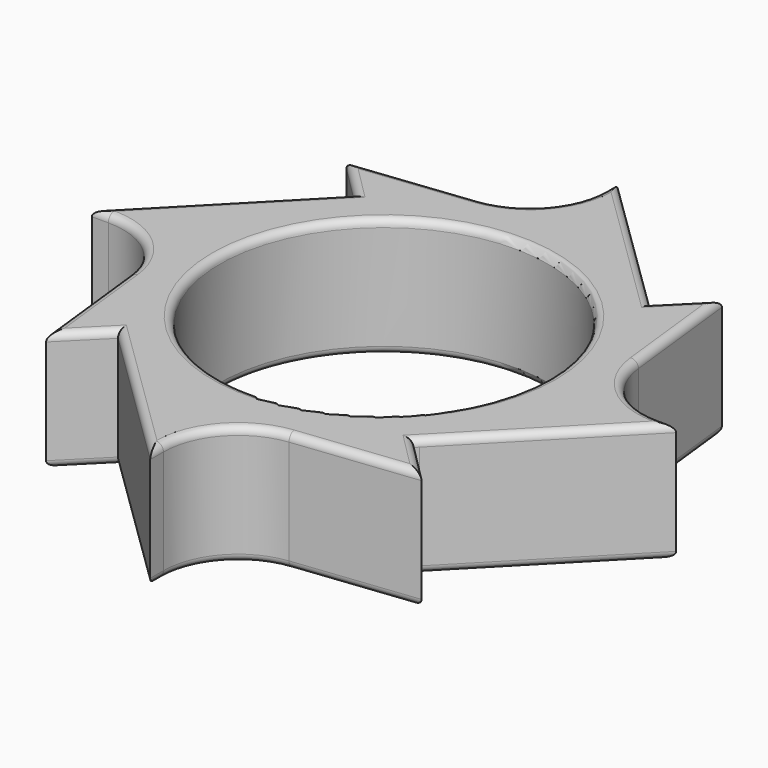
from build123d import *

# Parameters (mm, degrees)
F0_R          = 11
F1_DEPTH      = 8
F2_T1_DEPTH   = 2.3595992042
F2_T3_DEPTH   = 9.4400822056
F2_T5_DEPTH   = 2.3595992042
F2_T7_DEPTH   = 9.4400822056
F2_T9_DEPTH   = 2.3595992042
F2_T11_DEPTH  = 9.4400822056
F2_T13_DEPTH  = 2.3595992042
F2_T15_DEPTH  = 9.4400822056
F2_T18_ANGLE  = 83.5348176594
F2_T22_DEPTH  = 6.2837355468
F2_T27_DEPTH  = 16.3425213827
F2_T30_ANGLE  = 83.5348176594
F2_T34_DEPTH  = 6.2837355468
F2_T39_DEPTH  = 16.3425213827
F2_T42_ANGLE  = 83.5348176594
F2_T46_DEPTH  = 6.2837355468
F2_T51_DEPTH  = 16.3425213827
F2_T54_ANGLE  = 83.5348176594
F2_T58_DEPTH  = 6.2837355468
F2_T63_DEPTH  = 16.3425213827
F2_T68_ANGLE  = 83.5348176594
F2_T72_DEPTH  = 6.2837355468
F2_T77_DEPTH  = 16.3425213827
F2_T80_ANGLE  = 83.5348176594
F2_T84_DEPTH  = 6.2837355468
F2_T89_DEPTH  = 16.3425213827
F2_T92_ANGLE  = 83.5348176594
F2_T96_DEPTH  = 6.2837355468
F2_T101_DEPTH = 16.3425213827
F2_T104_ANGLE = 83.5348176594
F2_T108_DEPTH = 6.2837355468
F2_T113_DEPTH = 16.3425213827
F2_T121_DEPTH = 6.2837355468
F2_T125_DEPTH = 16.3425213827
F2_T132_DEPTH = 6.2837355468
F2_T136_DEPTH = 16.3425213827
F2_T143_DEPTH = 6.2837355468
F2_T147_DEPTH = 16.3425213827
F2_T154_DEPTH = 6.2837355468
F2_T158_DEPTH = 16.3425213827
F2_T165_DEPTH = 6.2837355468
F2_T169_DEPTH = 16.3425213827
F2_T176_DEPTH = 6.2837355468
F2_T180_DEPTH = 16.3425213827
F2_T187_DEPTH = 6.2837355468
F2_T191_DEPTH = 16.3425213827
F2_T198_DEPTH = 6.2837355468
F2_T202_DEPTH = 16.3425213827


# Not quite as in the source:
# - a fillet or chamfer that OpenCascade refuses, or shapes differently, is made with other operations: its cross-section is extruded or revolved along the edge and cut away or added


with BuildPart() as f1:
    # F0 (on Top) → F1 (new body)
    with BuildSketch(Plane.XY):
        with BuildLine():
            ThreePointArc((-85.174923351, 55.6713247205), (-75.4356150274, 59.7709133342), (-65.6050487553, 55.8952559455))
            Line((-65.6050487553, 55.8952559455), (-75.2754284143, 65.3468297839))
            Line((-75.2754284143, 65.3468297839), (-75.2754284143, 64.2372305797))
            ThreePointArc((-75.2754284143, 64.2372305797), (-76.5461533233, 60.9066889878), (-79.7124313324, 59.2690282604))
            Line((-79.7124313324, 59.2690282604), (-87.8504284143, 58.3468297839))
            Line((-87.8504284143, 58.3468297839), (-85.174923351, 55.6713247205))
        make_face()
        with BuildLine():
            ThreePointArc((-65.3759334777, 55.6713247205), (-62.3411149592, 51.129397837), (-61.2754284143, 45.7718297839))
            ThreePointArc((-61.2754284143, 45.7718297839), (-62.2806608854, 40.5626055741), (-65.1520022527, 36.1014501249))
            Line((-65.1520022527, 36.1014501249), (-55.7004284143, 45.7718297839))
            Line((-55.7004284143, 45.7718297839), (-56.8100276185, 45.7718297839))
            ThreePointArc((-56.8100276185, 45.7718297839), (-60.1405692104, 47.0425546929), (-61.7782299379, 50.208832702))
            Line((-61.7782299379, 50.208832702), (-62.7004284143, 58.3468297839))
            Line((-62.7004284143, 58.3468297839), (-65.3759334777, 55.6713247205))
        make_face()
        with BuildLine():
            Line((-62.7004284143, 33.1968297839), (-65.3759334777, 35.8723348473))
            ThreePointArc((-65.3759334777, 35.8723348473), (-75.1152418013, 31.7727462336), (-84.9458080734, 35.6484036223))
            Line((-84.9458080734, 35.6484036223), (-75.2754284143, 26.1968297839))
            Line((-75.2754284143, 26.1968297839), (-75.2754284143, 27.3064289881))
            ThreePointArc((-75.2754284143, 27.3064289881), (-74.0047035054, 30.63697058), (-70.8384254963, 32.2746313074))
            Line((-70.8384254963, 32.2746313074), (-62.7004284143, 33.1968297839))
        make_face()
        with BuildLine():
            ThreePointArc((-85.174923351, 35.8723348473), (-89.2745119647, 45.6116431709), (-85.398854576, 55.442209443))
            Line((-85.398854576, 55.442209443), (-94.8504284143, 45.7718297839))
            Line((-94.8504284143, 45.7718297839), (-93.7408292102, 45.7718297839))
            ThreePointArc((-93.7408292102, 45.7718297839), (-90.4102876183, 44.501104875), (-88.7726268908, 41.3348268658))
            Line((-88.7726268908, 41.3348268658), (-87.8504284143, 33.1968297839))
            Line((-87.8504284143, 33.1968297839), (-85.174923351, 35.8723348473))
        make_face()
        with BuildLine():
            ThreePointArc((-65.1520022527, 36.1014501249), (-62.2806608854, 40.5626055741), (-61.2754284143, 45.7718297839))
            ThreePointArc((-61.2754284143, 45.7718297839), (-62.3411149592, 51.129397837), (-65.3759334777, 55.6713247205))
            Line((-65.3759334777, 55.6713247205), (-65.6050487553, 55.8952559455))
            ThreePointArc((-65.6050487553, 55.8952559455), (-75.4356150274, 59.7709133342), (-85.174923351, 55.6713247205))
            Line((-85.174923351, 55.6713247205), (-85.398854576, 55.442209443))
            ThreePointArc((-85.398854576, 55.442209443), (-89.2745119647, 45.6116431709), (-85.174923351, 35.8723348473))
            Line((-85.174923351, 35.8723348473), (-84.9458080734, 35.6484036223))
            ThreePointArc((-84.9458080734, 35.6484036223), (-75.1152418013, 31.7727462336), (-65.3759334777, 35.8723348473))
            Line((-65.3759334777, 35.8723348473), (-65.1520022527, 36.1014501249))
        make_face()
        with Locations((-75.2754284143, 45.7718297839)):
            Circle(F0_R, mode=Mode.SUBTRACT)
    extrude(amount=F1_DEPTH)

    # F2: fillet of radius 0.5 on 42 edges, made by hand

    # F2_s2 → F2_t1 (cut)
    with BuildSketch(Plane.XZ.offset(-66.5968297839)):
        with BuildLine():
            ThreePointArc((-75.2754284143, 7.5), (-75.1289818049, 7.8535533906), (-74.7754284143, 8))
            Line((-74.7754284143, 8), (-75.2754284143, 8))
            Line((-75.2754284143, 8), (-75.2754284143, 7.5))
        make_face()
        with BuildLine():
            ThreePointArc((-75.2754284143, 0.5), (-75.1289818049, 0.1464466094), (-74.7754284143, 0))
            Line((-74.7754284143, 0), (-75.2754284143, 0))
            Line((-75.2754284143, 0), (-75.2754284143, 0.5))
        make_face()
    extrude(amount=F2_T1_DEPTH, mode=Mode.SUBTRACT)

    # F2_s4 → F2_t3 (cut)
    with BuildSketch(Plane(origin=(-72.0705704007, -8.1670427691, 0), x_dir=(0, 0, 1), z_dir=(-0.9936404639, -0.1125994164, 0))):
        with BuildLine():
            ThreePointArc((7.5, 67.86767798), (7.8535533906, 67.7212313705), (8, 67.36767798))
            Line((8, 67.36767798), (8, 67.86767798))
            Line((8, 67.86767798), (7.5, 67.86767798))
        make_face()
        with BuildLine():
            ThreePointArc((0.5, 67.86767798), (0.1464466094, 67.7212313705), (0, 67.36767798))
            Line((0, 67.36767798), (0, 67.86767798))
            Line((0, 67.86767798), (0.5, 67.86767798))
        make_face()
    extrude(amount=F2_T3_DEPTH, mode=Mode.SUBTRACT)

    # F2_s6 → F2_t5 (cut)
    with BuildSketch(Plane.YZ.offset(-96.1004284143)):
        with BuildLine():
            ThreePointArc((45.7718297839, 7.5), (45.9182763933, 7.8535533906), (46.2718297839, 8))
            Line((46.2718297839, 8), (45.7718297839, 8))
            Line((45.7718297839, 8), (45.7718297839, 7.5))
        make_face()
        with BuildLine():
            ThreePointArc((45.7718297839, 0.5), (45.9182763933, 0.1464466094), (46.2718297839, 0))
            Line((46.2718297839, 0), (45.7718297839, 0))
            Line((45.7718297839, 0), (45.7718297839, 0.5))
        make_face()
    extrude(amount=F2_T5_DEPTH, mode=Mode.SUBTRACT)

    # F2_s8 → F2_t7 (cut)
    with BuildSketch(Plane(origin=(-5.7501934997, 50.7429356199, 0), x_dir=(0, 0, 1), z_dir=(0.1125994164, -0.9936404639, 0))):
        with BuildLine():
            ThreePointArc((7.5, 83.553796781), (7.8535533906, 83.4073501716), (8, 83.053796781))
            Line((8, 83.053796781), (8, 83.553796781))
            Line((8, 83.553796781), (7.5, 83.553796781))
        make_face()
        with BuildLine():
            ThreePointArc((0.5, 83.553796781), (0.1464466094, 83.4073501716), (0, 83.053796781))
            Line((0, 83.053796781), (0, 83.553796781))
            Line((0, 83.553796781), (0.5, 83.553796781))
        make_face()
    extrude(amount=F2_T7_DEPTH, mode=Mode.SUBTRACT)

    # F2_s10 → F2_t9 (cut)
    with BuildSketch(Plane.XZ.offset(-27.3064289881)):
        with BuildLine():
            ThreePointArc((-75.2754284143, 7.5), (-75.4218750238, 7.8535533906), (-75.7754284143, 8))
            Line((-75.7754284143, 8), (-75.2754284143, 8))
            Line((-75.2754284143, 8), (-75.2754284143, 7.5))
        make_face()
        with BuildLine():
            ThreePointArc((-75.2754284143, 0.5), (-75.4218750238, 0.1464466094), (-75.7754284143, 0))
            Line((-75.7754284143, 0), (-75.2754284143, 0))
            Line((-75.2754284143, 0), (-75.2754284143, 0.5))
        make_face()
    extrude(amount=F2_T9_DEPTH, mode=Mode.SUBTRACT)

    # F2_s12 → F2_t11 (cut)
    with BuildSketch(Plane(origin=(-66.3292979816, -7.516441322, 0), x_dir=(0, 0, 1), z_dir=(0.9936404639, 0.1125994164, 0))):
        with BuildLine():
            ThreePointArc((7.5, -40.0457449917), (7.8535533906, -40.1921916011), (8, -40.5457449917))
            Line((8, -40.5457449917), (8, -40.0457449917))
            Line((8, -40.0457449917), (7.5, -40.0457449917))
        make_face()
        with BuildLine():
            ThreePointArc((0.5, -40.0457449917), (0.1464466094, -40.1921916011), (0, -40.5457449917))
            Line((0, -40.5457449917), (0, -40.0457449917))
            Line((0, -40.0457449917), (0.5, -40.0457449917))
        make_face()
    extrude(amount=F2_T11_DEPTH, mode=Mode.SUBTRACT)

    # F2_s14 → F2_t13 (cut)
    with BuildSketch(Plane.YZ.offset(-56.8100276185)):
        with BuildLine():
            ThreePointArc((45.7718297839, 7.5), (45.6253831745, 7.8535533906), (45.2718297839, 8))
            Line((45.2718297839, 8), (45.7718297839, 8))
            Line((45.7718297839, 8), (45.7718297839, 7.5))
        make_face()
        with BuildLine():
            ThreePointArc((45.7718297839, 0.5), (45.6253831745, 0.1464466094), (45.2718297839, 0))
            Line((45.2718297839, 0), (45.7718297839, 0))
            Line((45.7718297839, 0), (45.7718297839, 0.5))
        make_face()
    extrude(amount=F2_T13_DEPTH, mode=Mode.SUBTRACT)

    # F2_s16 → F2_t15 (cut)
    with BuildSketch(Plane(origin=(-6.4007949468, 56.484208039, 0), x_dir=(0, 0, 1), z_dir=(-0.1125994164, 0.9936404639, 0))):
        with BuildLine():
            ThreePointArc((7.5, -55.7318637928), (7.8535533906, -55.8783104022), (8, -56.2318637928))
            Line((8, -56.2318637928), (8, -55.7318637928))
            Line((8, -55.7318637928), (7.5, -55.7318637928))
        make_face()
        with BuildLine():
            ThreePointArc((0.5, -55.7318637928), (0.1464466094, -55.8783104022), (0, -56.2318637928))
            Line((0, -56.2318637928), (0, -55.7318637928))
            Line((0, -55.7318637928), (0.5, -55.7318637928))
        make_face()
    extrude(amount=F2_T15_DEPTH, mode=Mode.SUBTRACT)

    # F2_s17 → F2_t18 (revolve, cut)
    with BuildSketch(Plane.XZ.offset(-64.2372305797)):
        with BuildLine():
            ThreePointArc((-75.2754284143, 7.5), (-75.1289818049, 7.8535533906), (-74.7754284143, 8))
            Line((-74.7754284143, 8), (-75.2754284143, 8))
            Line((-75.2754284143, 8), (-75.2754284143, 7.5))
        make_face()
    revolve(axis=Axis((-80.2754284143, 64.2372305797, 8), (0, 0, -1)), revolution_arc=F2_T18_ANGLE, mode=Mode.SUBTRACT)


with BuildPart() as f2_tool20:
    # F2_s21 → F2_t22 (new body)
    with BuildSketch(Plane(origin=(-73.9825125756, 73.9825125756, 0), x_dir=(0, 0, 1), z_dir=(0.7071067812, -0.7071067812, 0))):
        with BuildLine():
            ThreePointArc((7.5, 20.862194661), (7.8535533906, 20.7157480516), (8, 20.362194661))
            Line((8, 20.362194661), (8, 20.862194661))
            Line((8, 20.862194661), (7.5, 20.862194661))
        make_face()
    extrude(amount=F2_T22_DEPTH)

    split(bisect_by=Plane(origin=(-71.3903349466, 69.7750290975, 0), x_dir=(0, 0, 1), z_dir=(-0.7151511392, 0.6989698478, 0)), keep=Keep.TOP)


with BuildPart() as f1_1:
    add(f1.part)

    # F2_t19: cut F2_tool20
    add(f2_tool20.part, mode=Mode.SUBTRACT)


with BuildPart() as f2_tool25:
    # F2_s26 → F2_t27 (new body)
    with BuildSketch(Plane(origin=(-12.9108760947, -13.209765453, 0), x_dir=(0, 0, 1), z_dir=(-0.6989698478, -0.7151511392, 0))):
        with BuildLine():
            ThreePointArc((7.5, 99.8255208318), (7.8535533906, 99.6790742224), (8, 99.3255208318))
            Line((8, 99.3255208318), (8, 99.8255208318))
            Line((8, 99.8255208318), (7.5, 99.8255208318))
        make_face()
    extrude(amount=F2_T27_DEPTH)

    split(bisect_by=Plane(origin=(-14.7517993152, -14.7517993152, 0), x_dir=(0, 0, 1), z_dir=(-0.7071067812, -0.7071067812, 0)), keep=Keep.TOP)


with BuildPart() as f1_2:
    add(f1_1.part)

    # F2_t24: cut F2_tool25
    add(f2_tool25.part, mode=Mode.SUBTRACT)

    # F2_s29 → F2_t30 (revolve, cut)
    with BuildSketch(Plane.YZ.offset(-93.7408292102)):
        with BuildLine():
            ThreePointArc((45.7718297839, 7.5), (45.9182763933, 7.8535533906), (46.2718297839, 8))
            Line((46.2718297839, 8), (45.7718297839, 8))
            Line((45.7718297839, 8), (45.7718297839, 7.5))
        make_face()
    revolve(axis=Axis((-93.7408292102, 40.7718297839, 8), (0, 0, -1)), revolution_arc=F2_T30_ANGLE, mode=Mode.SUBTRACT)


with BuildPart() as f2_tool32:
    # F2_s33 → F2_t34 (new body)
    with BuildSketch(Plane(origin=(-28.2106827917, -28.2106827917, 0), x_dir=(0, 0, 1), z_dir=(0.7071067812, 0.7071067812, 0))):
        with BuildLine():
            ThreePointArc((7.5, -85.593337116), (7.8535533906, -85.7397837254), (8, -86.093337116))
            Line((8, -86.093337116), (8, -85.593337116))
            Line((8, -85.593337116), (7.5, -85.593337116))
        make_face()
    extrude(amount=F2_T34_DEPTH)

    split(bisect_by=Plane(origin=(-23.6814913147, -24.2297225649, 0), x_dir=(0, 0, 1), z_dir=(-0.6989698478, -0.7151511392, 0)), keep=Keep.TOP)


with BuildPart() as f1_3:
    add(f1_2.part)

    # F2_t31: cut F2_tool32
    add(f2_tool32.part, mode=Mode.SUBTRACT)


with BuildPart() as f2_tool37:
    # F2_s38 → F2_t39 (new body)
    with BuildSketch(Plane(origin=(-62.3873709603, 60.9757697219, 0), x_dir=(0, 0, 1), z_dir=(0.7151511392, -0.6989698478, 0))):
        with BuildLine():
            ThreePointArc((7.5, 33.8805620741), (7.8535533906, 33.7341154647), (8, 33.3805620741))
            Line((8, 33.3805620741), (8, 33.8805620741))
            Line((8, 33.8805620741), (7.5, 33.8805620741))
        make_face()
    extrude(amount=F2_T39_DEPTH)

    split(bisect_by=Plane(origin=(-60.5236290991, 60.5236290991, 0), x_dir=(0, 0, 1), z_dir=(0.7071067812, -0.7071067812, 0)), keep=Keep.TOP)


with BuildPart() as f1_4:
    add(f1_3.part)

    # F2_t36: cut F2_tool37
    add(f2_tool37.part, mode=Mode.SUBTRACT)

    # F2_s41 → F2_t42 (revolve, cut)
    with BuildSketch(Plane.XZ.offset(-27.3064289881)):
        with BuildLine():
            ThreePointArc((-75.2754284143, 7.5), (-75.4218750238, 7.8535533906), (-75.7754284143, 8))
            Line((-75.7754284143, 8), (-75.2754284143, 8))
            Line((-75.2754284143, 8), (-75.2754284143, 7.5))
        make_face()
    revolve(axis=Axis((-70.2754284143, 27.3064289881, 8), (0, 0, -1)), revolution_arc=F2_T42_ANGLE, mode=Mode.SUBTRACT)


with BuildPart() as f2_tool44:
    # F2_s45 → F2_t46 (new body)
    with BuildSketch(Plane(origin=(-47.0647456226, 47.0647456226, 0), x_dir=(0, 0, 1), z_dir=(-0.7071067812, 0.7071067812, 0))):
        with BuildLine():
            ThreePointArc((7.5, -20.862194661), (7.8535533906, -21.0086412704), (8, -21.362194661))
            Line((8, -21.362194661), (8, -20.862194661))
            Line((8, -20.862194661), (7.5, -20.862194661))
        make_face()
    extrude(amount=F2_T46_DEPTH)

    split(bisect_by=Plane(origin=(-51.3674138484, 50.2051545019, 0), x_dir=(0, 0, 1), z_dir=(0.7151511392, -0.6989698478, 0)), keep=Keep.TOP)


with BuildPart() as f1_5:
    add(f1_4.part)

    # F2_t43: cut F2_tool44
    add(f2_tool44.part, mode=Mode.SUBTRACT)


with BuildPart() as f2_tool49:
    # F2_s50 → F2_t51 (new body)
    with BuildSketch(Plane(origin=(-14.8822319391, -15.2267585786, 0), x_dir=(0, 0, 1), z_dir=(0.6989698478, 0.7151511392, 0))):
        with BuildLine():
            ThreePointArc((7.5, -71.8273537312), (7.8535533906, -71.9738003406), (8, -72.3273537312))
            Line((8, -72.3273537312), (8, -71.8273537312))
            Line((8, -71.8273537312), (7.5, -71.8273537312))
        make_face()
    extrude(amount=F2_T51_DEPTH)

    split(bisect_by=Plane(origin=(-14.7517993152, -14.7517993152, 0), x_dir=(0, 0, 1), z_dir=(0.7071067812, 0.7071067812, 0)), keep=Keep.TOP)


with BuildPart() as f1_6:
    add(f1_5.part)

    # F2_t48: cut F2_tool49
    add(f2_tool49.part, mode=Mode.SUBTRACT)

    # F2_s53 → F2_t54 (revolve, cut)
    with BuildSketch(Plane.YZ.offset(-56.8100276185)):
        with BuildLine():
            ThreePointArc((45.7718297839, 7.5), (45.6253831745, 7.8535533906), (45.2718297839, 8))
            Line((45.2718297839, 8), (45.7718297839, 8))
            Line((45.7718297839, 8), (45.7718297839, 7.5))
        make_face()
    revolve(axis=Axis((-56.8100276185, 50.7718297839, 8), (0, 0, -1)), revolution_arc=F2_T54_ANGLE, mode=Mode.SUBTRACT)


with BuildPart() as f2_tool56:
    # F2_s57 → F2_t58 (new body)
    with BuildSketch(Plane(origin=(-1.2929158387, -1.2929158387, 0), x_dir=(0, 0, 1), z_dir=(-0.7071067812, -0.7071067812, 0))):
        with BuildLine():
            ThreePointArc((7.5, 85.593337116), (7.8535533906, 85.4468905066), (8, 85.093337116))
            Line((8, 85.093337116), (8, 85.593337116))
            Line((8, 85.593337116), (7.5, 85.593337116))
        make_face()
    extrude(amount=F2_T58_DEPTH)

    split(bisect_by=Plane(origin=(-4.111616719, -4.2068014667, 0), x_dir=(0, 0, 1), z_dir=(0.6989698478, 0.7151511392, 0)), keep=Keep.TOP)


with BuildPart() as f1_7:
    add(f1_6.part)

    # F2_t55: cut F2_tool56
    add(f2_tool56.part, mode=Mode.SUBTRACT)


with BuildPart() as f2_tool61:
    # F2_s62 → F2_t63 (new body)
    with BuildSketch(Plane(origin=(-60.3703778347, 59.0044138775, 0), x_dir=(0, 0, 1), z_dir=(-0.7151511392, 0.6989698478, 0))):
        with BuildLine():
            ThreePointArc((7.5, -5.8823949735), (7.8535533906, -6.0288415829), (8, -6.3823949735))
            Line((8, -6.3823949735), (8, -5.8823949735))
            Line((8, -5.8823949735), (7.5, -5.8823949735))
        make_face()
    extrude(amount=F2_T63_DEPTH)

    split(bisect_by=Plane(origin=(-60.5236290991, 60.5236290991, 0), x_dir=(0, 0, 1), z_dir=(-0.7071067812, 0.7071067812, 0)), keep=Keep.TOP)


with BuildPart() as f1_8:
    add(f1_7.part)

    # F2_t60: cut F2_tool61
    add(f2_tool61.part, mode=Mode.SUBTRACT)

    # F2_s65 → F2_t66 (revolve, cut)
    with BuildSketch(Plane.XZ.offset(-45.7718297839)):
        with BuildLine():
            ThreePointArc((-64.2754284143, 7.5), (-64.1289818049, 7.8535533906), (-63.7754284143, 8))
            Line((-63.7754284143, 8), (-64.2754284143, 8))
            Line((-64.2754284143, 8), (-64.2754284143, 7.5))
        make_face()
    revolve(axis=Axis((-75.2754284143, 45.7718297839, 8), (0, 0, 1)), mode=Mode.SUBTRACT)

    # F2_s67 → F2_t68 (revolve, cut)
    with BuildSketch(Plane.XZ.offset(-64.2372305797)):
        with BuildLine():
            ThreePointArc((-75.2754284143, 0.5), (-75.1289818049, 0.1464466094), (-74.7754284143, 0))
            Line((-74.7754284143, 0), (-75.2754284143, 0))
            Line((-75.2754284143, 0), (-75.2754284143, 0.5))
        make_face()
    revolve(axis=Axis((-80.2754284143, 64.2372305797, 0), (0, 0, -1)), revolution_arc=F2_T68_ANGLE, mode=Mode.SUBTRACT)


with BuildPart() as f2_tool70:
    # F2_s71 → F2_t72 (new body)
    with BuildSketch(Plane(origin=(-73.9825125756, 73.9825125756, 0), x_dir=(0, 0, 1), z_dir=(0.7071067812, -0.7071067812, 0))):
        with BuildLine():
            ThreePointArc((0.5, 20.862194661), (0.1464466094, 20.7157480516), (0, 20.362194661))
            Line((0, 20.362194661), (0, 20.862194661))
            Line((0, 20.862194661), (0.5, 20.862194661))
        make_face()
    extrude(amount=F2_T72_DEPTH)

    split(bisect_by=Plane(origin=(-71.3903349466, 69.7750290975, 0), x_dir=(0, 0, 1), z_dir=(-0.7151511392, 0.6989698478, 0)), keep=Keep.TOP)


with BuildPart() as f1_9:
    add(f1_8.part)

    # F2_t69: cut F2_tool70
    add(f2_tool70.part, mode=Mode.SUBTRACT)


with BuildPart() as f2_tool75:
    # F2_s76 → F2_t77 (new body)
    with BuildSketch(Plane(origin=(-12.9108760947, -13.209765453, 0), x_dir=(0, 0, 1), z_dir=(-0.6989698478, -0.7151511392, 0))):
        with BuildLine():
            ThreePointArc((0.5, 99.8255208318), (0.1464466094, 99.6790742224), (0, 99.3255208318))
            Line((0, 99.3255208318), (0, 99.8255208318))
            Line((0, 99.8255208318), (0.5, 99.8255208318))
        make_face()
    extrude(amount=F2_T77_DEPTH)

    split(bisect_by=Plane(origin=(-14.7517993152, -14.7517993152, 0), x_dir=(0, 0, 1), z_dir=(-0.7071067812, -0.7071067812, 0)), keep=Keep.TOP)


with BuildPart() as f1_10:
    add(f1_9.part)

    # F2_t74: cut F2_tool75
    add(f2_tool75.part, mode=Mode.SUBTRACT)

    # F2_s79 → F2_t80 (revolve, cut)
    with BuildSketch(Plane.YZ.offset(-93.7408292102)):
        with BuildLine():
            ThreePointArc((45.7718297839, 0.5), (45.9182763933, 0.1464466094), (46.2718297839, 0))
            Line((46.2718297839, 0), (45.7718297839, 0))
            Line((45.7718297839, 0), (45.7718297839, 0.5))
        make_face()
    revolve(axis=Axis((-93.7408292102, 40.7718297839, 0), (0, 0, -1)), revolution_arc=F2_T80_ANGLE, mode=Mode.SUBTRACT)


with BuildPart() as f2_tool82:
    # F2_s83 → F2_t84 (new body)
    with BuildSketch(Plane(origin=(-28.2106827917, -28.2106827917, 0), x_dir=(0, 0, 1), z_dir=(0.7071067812, 0.7071067812, 0))):
        with BuildLine():
            ThreePointArc((0.5, -85.593337116), (0.1464466094, -85.7397837254), (0, -86.093337116))
            Line((0, -86.093337116), (0, -85.593337116))
            Line((0, -85.593337116), (0.5, -85.593337116))
        make_face()
    extrude(amount=F2_T84_DEPTH)

    split(bisect_by=Plane(origin=(-23.6814913147, -24.2297225649, 0), x_dir=(0, 0, 1), z_dir=(-0.6989698478, -0.7151511392, 0)), keep=Keep.TOP)


with BuildPart() as f1_11:
    add(f1_10.part)

    # F2_t81: cut F2_tool82
    add(f2_tool82.part, mode=Mode.SUBTRACT)


with BuildPart() as f2_tool87:
    # F2_s88 → F2_t89 (new body)
    with BuildSketch(Plane(origin=(-62.3873709603, 60.9757697219, 0), x_dir=(0, 0, 1), z_dir=(0.7151511392, -0.6989698478, 0))):
        with BuildLine():
            ThreePointArc((0.5, 33.8805620741), (0.1464466094, 33.7341154647), (0, 33.3805620741))
            Line((0, 33.3805620741), (0, 33.8805620741))
            Line((0, 33.8805620741), (0.5, 33.8805620741))
        make_face()
    extrude(amount=F2_T89_DEPTH)

    split(bisect_by=Plane(origin=(-60.5236290991, 60.5236290991, 0), x_dir=(0, 0, 1), z_dir=(0.7071067812, -0.7071067812, 0)), keep=Keep.TOP)


with BuildPart() as f1_12:
    add(f1_11.part)

    # F2_t86: cut F2_tool87
    add(f2_tool87.part, mode=Mode.SUBTRACT)

    # F2_s91 → F2_t92 (revolve, cut)
    with BuildSketch(Plane.XZ.offset(-27.3064289881)):
        with BuildLine():
            ThreePointArc((-75.2754284143, 0.5), (-75.4218750238, 0.1464466094), (-75.7754284143, 0))
            Line((-75.7754284143, 0), (-75.2754284143, 0))
            Line((-75.2754284143, 0), (-75.2754284143, 0.5))
        make_face()
    revolve(axis=Axis((-70.2754284143, 27.3064289881, 0), (0, 0, -1)), revolution_arc=F2_T92_ANGLE, mode=Mode.SUBTRACT)


with BuildPart() as f2_tool94:
    # F2_s95 → F2_t96 (new body)
    with BuildSketch(Plane(origin=(-47.0647456226, 47.0647456226, 0), x_dir=(0, 0, 1), z_dir=(-0.7071067812, 0.7071067812, 0))):
        with BuildLine():
            ThreePointArc((0.5, -20.862194661), (0.1464466094, -21.0086412704), (0, -21.362194661))
            Line((0, -21.362194661), (0, -20.862194661))
            Line((0, -20.862194661), (0.5, -20.862194661))
        make_face()
    extrude(amount=F2_T96_DEPTH)

    split(bisect_by=Plane(origin=(-51.3674138484, 50.2051545019, 0), x_dir=(0, 0, 1), z_dir=(0.7151511392, -0.6989698478, 0)), keep=Keep.TOP)


with BuildPart() as f1_13:
    add(f1_12.part)

    # F2_t93: cut F2_tool94
    add(f2_tool94.part, mode=Mode.SUBTRACT)


with BuildPart() as f2_tool99:
    # F2_s100 → F2_t101 (new body)
    with BuildSketch(Plane(origin=(-14.8822319391, -15.2267585786, 0), x_dir=(0, 0, 1), z_dir=(0.6989698478, 0.7151511392, 0))):
        with BuildLine():
            ThreePointArc((0.5, -71.8273537312), (0.1464466094, -71.9738003406), (0, -72.3273537312))
            Line((0, -72.3273537312), (0, -71.8273537312))
            Line((0, -71.8273537312), (0.5, -71.8273537312))
        make_face()
    extrude(amount=F2_T101_DEPTH)

    split(bisect_by=Plane(origin=(-14.7517993152, -14.7517993152, 0), x_dir=(0, 0, 1), z_dir=(0.7071067812, 0.7071067812, 0)), keep=Keep.TOP)


with BuildPart() as f1_14:
    add(f1_13.part)

    # F2_t98: cut F2_tool99
    add(f2_tool99.part, mode=Mode.SUBTRACT)

    # F2_s103 → F2_t104 (revolve, cut)
    with BuildSketch(Plane.YZ.offset(-56.8100276185)):
        with BuildLine():
            ThreePointArc((45.7718297839, 0.5), (45.6253831745, 0.1464466094), (45.2718297839, 0))
            Line((45.2718297839, 0), (45.7718297839, 0))
            Line((45.7718297839, 0), (45.7718297839, 0.5))
        make_face()
    revolve(axis=Axis((-56.8100276185, 50.7718297839, 0), (0, 0, -1)), revolution_arc=F2_T104_ANGLE, mode=Mode.SUBTRACT)


with BuildPart() as f2_tool106:
    # F2_s107 → F2_t108 (new body)
    with BuildSketch(Plane(origin=(-1.2929158387, -1.2929158387, 0), x_dir=(0, 0, 1), z_dir=(-0.7071067812, -0.7071067812, 0))):
        with BuildLine():
            ThreePointArc((0.5, 85.593337116), (0.1464466094, 85.4468905066), (0, 85.093337116))
            Line((0, 85.093337116), (0, 85.593337116))
            Line((0, 85.593337116), (0.5, 85.593337116))
        make_face()
    extrude(amount=F2_T108_DEPTH)

    split(bisect_by=Plane(origin=(-4.111616719, -4.2068014667, 0), x_dir=(0, 0, 1), z_dir=(0.6989698478, 0.7151511392, 0)), keep=Keep.TOP)


with BuildPart() as f1_15:
    add(f1_14.part)

    # F2_t105: cut F2_tool106
    add(f2_tool106.part, mode=Mode.SUBTRACT)


with BuildPart() as f2_tool111:
    # F2_s112 → F2_t113 (new body)
    with BuildSketch(Plane(origin=(-60.3703778347, 59.0044138775, 0), x_dir=(0, 0, 1), z_dir=(-0.7151511392, 0.6989698478, 0))):
        with BuildLine():
            ThreePointArc((0.5, -5.8823949735), (0.1464466094, -6.0288415829), (0, -6.3823949735))
            Line((0, -6.3823949735), (0, -5.8823949735))
            Line((0, -5.8823949735), (0.5, -5.8823949735))
        make_face()
    extrude(amount=F2_T113_DEPTH)

    split(bisect_by=Plane(origin=(-60.5236290991, 60.5236290991, 0), x_dir=(0, 0, 1), z_dir=(-0.7071067812, 0.7071067812, 0)), keep=Keep.TOP)


with BuildPart() as f1_16:
    add(f1_15.part)

    # F2_t110: cut F2_tool111
    add(f2_tool111.part, mode=Mode.SUBTRACT)

    # F2_s115 → F2_t116 (revolve, cut)
    with BuildSketch(Plane.XZ.offset(-45.7718297839)):
        with BuildLine():
            ThreePointArc((-64.2754284143, 0.5), (-64.1289818049, 0.1464466094), (-63.7754284143, 0))
            Line((-63.7754284143, 0), (-64.2754284143, 0))
            Line((-64.2754284143, 0), (-64.2754284143, 0.5))
        make_face()
    revolve(axis=Axis((-75.2754284143, 45.7718297839, 0), (0, 0, 1)), mode=Mode.SUBTRACT)


with BuildPart() as f2_tool119:
    # F2_s120 → F2_t121 (new body)
    with BuildSketch(Plane(origin=(-73.9825125756, 73.9825125756, 0), x_dir=(0, 0, 1), z_dir=(0.7071067812, -0.7071067812, 0))):
        with BuildLine():
            ThreePointArc((7.5, 20.862194661), (7.8535533906, 20.7157480516), (8, 20.362194661))
            Line((8, 20.362194661), (8, 20.862194661))
            Line((8, 20.862194661), (7.5, 20.862194661))
        make_face()
    extrude(amount=F2_T121_DEPTH)

    split(bisect_by=Plane(origin=(-71.3903349466, 69.7750290975, 0), x_dir=(0, 0, 1), z_dir=(0.7151511392, -0.6989698478, 0)), keep=Keep.TOP)


with BuildPart() as f2_tool123:
    # F2_s124 → F2_t125 (new body)
    with BuildSketch(Plane(origin=(-12.9108760947, -13.209765453, 0), x_dir=(0, 0, 1), z_dir=(-0.6989698478, -0.7151511392, 0))):
        with BuildLine():
            ThreePointArc((7.5, 99.8255208318), (7.8535533906, 99.6790742224), (8, 99.3255208318))
            Line((8, 99.3255208318), (8, 99.8255208318))
            Line((8, 99.8255208318), (7.5, 99.8255208318))
        make_face()
    extrude(amount=F2_T125_DEPTH)

    split(bisect_by=Plane(origin=(-14.7517993152, -14.7517993152, 0), x_dir=(0, 0, 1), z_dir=(0.7071067812, 0.7071067812, 0)), keep=Keep.TOP)


with BuildPart() as f2_tool119_1:
    add(f2_tool119.part)

    # F2_t127: intersect F2_tool123
    add(f2_tool123.part, mode=Mode.INTERSECT)


with BuildPart() as f1_17:
    add(f1_16.part)

    # F2_t117: cut F2_tool119
    add(f2_tool119_1.part, mode=Mode.SUBTRACT)


with BuildPart() as f2_tool130:
    # F2_s131 → F2_t132 (new body)
    with BuildSketch(Plane(origin=(-28.2106827917, -28.2106827917, 0), x_dir=(0, 0, 1), z_dir=(0.7071067812, 0.7071067812, 0))):
        with BuildLine():
            ThreePointArc((7.5, -85.593337116), (7.8535533906, -85.7397837254), (8, -86.093337116))
            Line((8, -86.093337116), (8, -85.593337116))
            Line((8, -85.593337116), (7.5, -85.593337116))
        make_face()
    extrude(amount=F2_T132_DEPTH)

    split(bisect_by=Plane(origin=(-23.6814913147, -24.2297225649, 0), x_dir=(0, 0, 1), z_dir=(0.6989698478, 0.7151511392, 0)), keep=Keep.TOP)


with BuildPart() as f2_tool134:
    # F2_s135 → F2_t136 (new body)
    with BuildSketch(Plane(origin=(-62.3873709603, 60.9757697219, 0), x_dir=(0, 0, 1), z_dir=(0.7151511392, -0.6989698478, 0))):
        with BuildLine():
            ThreePointArc((7.5, 33.8805620741), (7.8535533906, 33.7341154647), (8, 33.3805620741))
            Line((8, 33.3805620741), (8, 33.8805620741))
            Line((8, 33.8805620741), (7.5, 33.8805620741))
        make_face()
    extrude(amount=F2_T136_DEPTH)

    split(bisect_by=Plane(origin=(-60.5236290991, 60.5236290991, 0), x_dir=(0, 0, 1), z_dir=(-0.7071067812, 0.7071067812, 0)), keep=Keep.TOP)


with BuildPart() as f2_tool130_1:
    add(f2_tool130.part)

    # F2_t138: intersect F2_tool134
    add(f2_tool134.part, mode=Mode.INTERSECT)


with BuildPart() as f1_18:
    add(f1_17.part)

    # F2_t128: cut F2_tool130
    add(f2_tool130_1.part, mode=Mode.SUBTRACT)


with BuildPart() as f2_tool141:
    # F2_s142 → F2_t143 (new body)
    with BuildSketch(Plane(origin=(-47.0647456226, 47.0647456226, 0), x_dir=(0, 0, 1), z_dir=(-0.7071067812, 0.7071067812, 0))):
        with BuildLine():
            ThreePointArc((7.5, -20.862194661), (7.8535533906, -21.0086412704), (8, -21.362194661))
            Line((8, -21.362194661), (8, -20.862194661))
            Line((8, -20.862194661), (7.5, -20.862194661))
        make_face()
    extrude(amount=F2_T143_DEPTH)

    split(bisect_by=Plane(origin=(-51.3674138484, 50.2051545019, 0), x_dir=(0, 0, 1), z_dir=(-0.7151511392, 0.6989698478, 0)), keep=Keep.TOP)


with BuildPart() as f2_tool145:
    # F2_s146 → F2_t147 (new body)
    with BuildSketch(Plane(origin=(-14.8822319391, -15.2267585786, 0), x_dir=(0, 0, 1), z_dir=(0.6989698478, 0.7151511392, 0))):
        with BuildLine():
            ThreePointArc((7.5, -71.8273537312), (7.8535533906, -71.9738003406), (8, -72.3273537312))
            Line((8, -72.3273537312), (8, -71.8273537312))
            Line((8, -71.8273537312), (7.5, -71.8273537312))
        make_face()
    extrude(amount=F2_T147_DEPTH)

    split(bisect_by=Plane(origin=(-14.7517993152, -14.7517993152, 0), x_dir=(0, 0, 1), z_dir=(-0.7071067812, -0.7071067812, 0)), keep=Keep.TOP)


with BuildPart() as f2_tool141_1:
    add(f2_tool141.part)

    # F2_t149: intersect F2_tool145
    add(f2_tool145.part, mode=Mode.INTERSECT)


with BuildPart() as f1_19:
    add(f1_18.part)

    # F2_t139: cut F2_tool141
    add(f2_tool141_1.part, mode=Mode.SUBTRACT)


with BuildPart() as f2_tool152:
    # F2_s153 → F2_t154 (new body)
    with BuildSketch(Plane(origin=(-1.2929158387, -1.2929158387, 0), x_dir=(0, 0, 1), z_dir=(-0.7071067812, -0.7071067812, 0))):
        with BuildLine():
            ThreePointArc((7.5, 85.593337116), (7.8535533906, 85.4468905066), (8, 85.093337116))
            Line((8, 85.093337116), (8, 85.593337116))
            Line((8, 85.593337116), (7.5, 85.593337116))
        make_face()
    extrude(amount=F2_T154_DEPTH)

    split(bisect_by=Plane(origin=(-4.111616719, -4.2068014667, 0), x_dir=(0, 0, 1), z_dir=(-0.6989698478, -0.7151511392, 0)), keep=Keep.TOP)


with BuildPart() as f2_tool156:
    # F2_s157 → F2_t158 (new body)
    with BuildSketch(Plane(origin=(-60.3703778347, 59.0044138775, 0), x_dir=(0, 0, 1), z_dir=(-0.7151511392, 0.6989698478, 0))):
        with BuildLine():
            ThreePointArc((7.5, -5.8823949735), (7.8535533906, -6.0288415829), (8, -6.3823949735))
            Line((8, -6.3823949735), (8, -5.8823949735))
            Line((8, -5.8823949735), (7.5, -5.8823949735))
        make_face()
    extrude(amount=F2_T158_DEPTH)

    split(bisect_by=Plane(origin=(-60.5236290991, 60.5236290991, 0), x_dir=(0, 0, 1), z_dir=(0.7071067812, -0.7071067812, 0)), keep=Keep.TOP)


with BuildPart() as f2_tool152_1:
    add(f2_tool152.part)

    # F2_t160: intersect F2_tool156
    add(f2_tool156.part, mode=Mode.INTERSECT)


with BuildPart() as f1_20:
    add(f1_19.part)

    # F2_t150: cut F2_tool152
    add(f2_tool152_1.part, mode=Mode.SUBTRACT)


with BuildPart() as f2_tool163:
    # F2_s164 → F2_t165 (new body)
    with BuildSketch(Plane(origin=(-73.9825125756, 73.9825125756, 0), x_dir=(0, 0, 1), z_dir=(0.7071067812, -0.7071067812, 0))):
        with BuildLine():
            ThreePointArc((0.5, 20.862194661), (0.1464466094, 20.7157480516), (0, 20.362194661))
            Line((0, 20.362194661), (0, 20.862194661))
            Line((0, 20.862194661), (0.5, 20.862194661))
        make_face()
    extrude(amount=F2_T165_DEPTH)

    split(bisect_by=Plane(origin=(-71.3903349466, 69.7750290975, 0), x_dir=(0, 0, 1), z_dir=(0.7151511392, -0.6989698478, 0)), keep=Keep.TOP)


with BuildPart() as f2_tool167:
    # F2_s168 → F2_t169 (new body)
    with BuildSketch(Plane(origin=(-12.9108760947, -13.209765453, 0), x_dir=(0, 0, 1), z_dir=(-0.6989698478, -0.7151511392, 0))):
        with BuildLine():
            ThreePointArc((0.5, 99.8255208318), (0.1464466094, 99.6790742224), (0, 99.3255208318))
            Line((0, 99.3255208318), (0, 99.8255208318))
            Line((0, 99.8255208318), (0.5, 99.8255208318))
        make_face()
    extrude(amount=F2_T169_DEPTH)

    split(bisect_by=Plane(origin=(-14.7517993152, -14.7517993152, 0), x_dir=(0, 0, 1), z_dir=(0.7071067812, 0.7071067812, 0)), keep=Keep.TOP)


with BuildPart() as f2_tool163_1:
    add(f2_tool163.part)

    # F2_t171: intersect F2_tool167
    add(f2_tool167.part, mode=Mode.INTERSECT)


with BuildPart() as f1_21:
    add(f1_20.part)

    # F2_t161: cut F2_tool163
    add(f2_tool163_1.part, mode=Mode.SUBTRACT)


with BuildPart() as f2_tool174:
    # F2_s175 → F2_t176 (new body)
    with BuildSketch(Plane(origin=(-28.2106827917, -28.2106827917, 0), x_dir=(0, 0, 1), z_dir=(0.7071067812, 0.7071067812, 0))):
        with BuildLine():
            ThreePointArc((0.5, -85.593337116), (0.1464466094, -85.7397837254), (0, -86.093337116))
            Line((0, -86.093337116), (0, -85.593337116))
            Line((0, -85.593337116), (0.5, -85.593337116))
        make_face()
    extrude(amount=F2_T176_DEPTH)

    split(bisect_by=Plane(origin=(-23.6814913147, -24.2297225649, 0), x_dir=(0, 0, 1), z_dir=(0.6989698478, 0.7151511392, 0)), keep=Keep.TOP)


with BuildPart() as f2_tool178:
    # F2_s179 → F2_t180 (new body)
    with BuildSketch(Plane(origin=(-62.3873709603, 60.9757697219, 0), x_dir=(0, 0, 1), z_dir=(0.7151511392, -0.6989698478, 0))):
        with BuildLine():
            ThreePointArc((0.5, 33.8805620741), (0.1464466094, 33.7341154647), (0, 33.3805620741))
            Line((0, 33.3805620741), (0, 33.8805620741))
            Line((0, 33.8805620741), (0.5, 33.8805620741))
        make_face()
    extrude(amount=F2_T180_DEPTH)

    split(bisect_by=Plane(origin=(-60.5236290991, 60.5236290991, 0), x_dir=(0, 0, 1), z_dir=(-0.7071067812, 0.7071067812, 0)), keep=Keep.TOP)


with BuildPart() as f2_tool174_1:
    add(f2_tool174.part)

    # F2_t182: intersect F2_tool178
    add(f2_tool178.part, mode=Mode.INTERSECT)


with BuildPart() as f1_22:
    add(f1_21.part)

    # F2_t172: cut F2_tool174
    add(f2_tool174_1.part, mode=Mode.SUBTRACT)


with BuildPart() as f2_tool185:
    # F2_s186 → F2_t187 (new body)
    with BuildSketch(Plane(origin=(-47.0647456226, 47.0647456226, 0), x_dir=(0, 0, 1), z_dir=(-0.7071067812, 0.7071067812, 0))):
        with BuildLine():
            ThreePointArc((0.5, -20.862194661), (0.1464466094, -21.0086412704), (0, -21.362194661))
            Line((0, -21.362194661), (0, -20.862194661))
            Line((0, -20.862194661), (0.5, -20.862194661))
        make_face()
    extrude(amount=F2_T187_DEPTH)

    split(bisect_by=Plane(origin=(-51.3674138484, 50.2051545019, 0), x_dir=(0, 0, 1), z_dir=(-0.7151511392, 0.6989698478, 0)), keep=Keep.TOP)


with BuildPart() as f2_tool189:
    # F2_s190 → F2_t191 (new body)
    with BuildSketch(Plane(origin=(-14.8822319391, -15.2267585786, 0), x_dir=(0, 0, 1), z_dir=(0.6989698478, 0.7151511392, 0))):
        with BuildLine():
            ThreePointArc((0.5, -71.8273537312), (0.1464466094, -71.9738003406), (0, -72.3273537312))
            Line((0, -72.3273537312), (0, -71.8273537312))
            Line((0, -71.8273537312), (0.5, -71.8273537312))
        make_face()
    extrude(amount=F2_T191_DEPTH)

    split(bisect_by=Plane(origin=(-14.7517993152, -14.7517993152, 0), x_dir=(0, 0, 1), z_dir=(-0.7071067812, -0.7071067812, 0)), keep=Keep.TOP)


with BuildPart() as f2_tool185_1:
    add(f2_tool185.part)

    # F2_t193: intersect F2_tool189
    add(f2_tool189.part, mode=Mode.INTERSECT)


with BuildPart() as f1_23:
    add(f1_22.part)

    # F2_t183: cut F2_tool185
    add(f2_tool185_1.part, mode=Mode.SUBTRACT)


with BuildPart() as f2_tool196:
    # F2_s197 → F2_t198 (new body)
    with BuildSketch(Plane(origin=(-1.2929158387, -1.2929158387, 0), x_dir=(0, 0, 1), z_dir=(-0.7071067812, -0.7071067812, 0))):
        with BuildLine():
            ThreePointArc((0.5, 85.593337116), (0.1464466094, 85.4468905066), (0, 85.093337116))
            Line((0, 85.093337116), (0, 85.593337116))
            Line((0, 85.593337116), (0.5, 85.593337116))
        make_face()
    extrude(amount=F2_T198_DEPTH)

    split(bisect_by=Plane(origin=(-4.111616719, -4.2068014667, 0), x_dir=(0, 0, 1), z_dir=(-0.6989698478, -0.7151511392, 0)), keep=Keep.TOP)


with BuildPart() as f2_tool200:
    # F2_s201 → F2_t202 (new body)
    with BuildSketch(Plane(origin=(-60.3703778347, 59.0044138775, 0), x_dir=(0, 0, 1), z_dir=(-0.7151511392, 0.6989698478, 0))):
        with BuildLine():
            ThreePointArc((0.5, -5.8823949735), (0.1464466094, -6.0288415829), (0, -6.3823949735))
            Line((0, -6.3823949735), (0, -5.8823949735))
            Line((0, -5.8823949735), (0.5, -5.8823949735))
        make_face()
    extrude(amount=F2_T202_DEPTH)

    split(bisect_by=Plane(origin=(-60.5236290991, 60.5236290991, 0), x_dir=(0, 0, 1), z_dir=(0.7071067812, -0.7071067812, 0)), keep=Keep.TOP)


with BuildPart() as f2_tool196_1:
    add(f2_tool196.part)

    # F2_t204: intersect F2_tool200
    add(f2_tool200.part, mode=Mode.INTERSECT)


with BuildPart() as f1_24:
    add(f1_23.part)

    # F2_t194: cut F2_tool196
    add(f2_tool196_1.part, mode=Mode.SUBTRACT)


solid = f1_24.part
